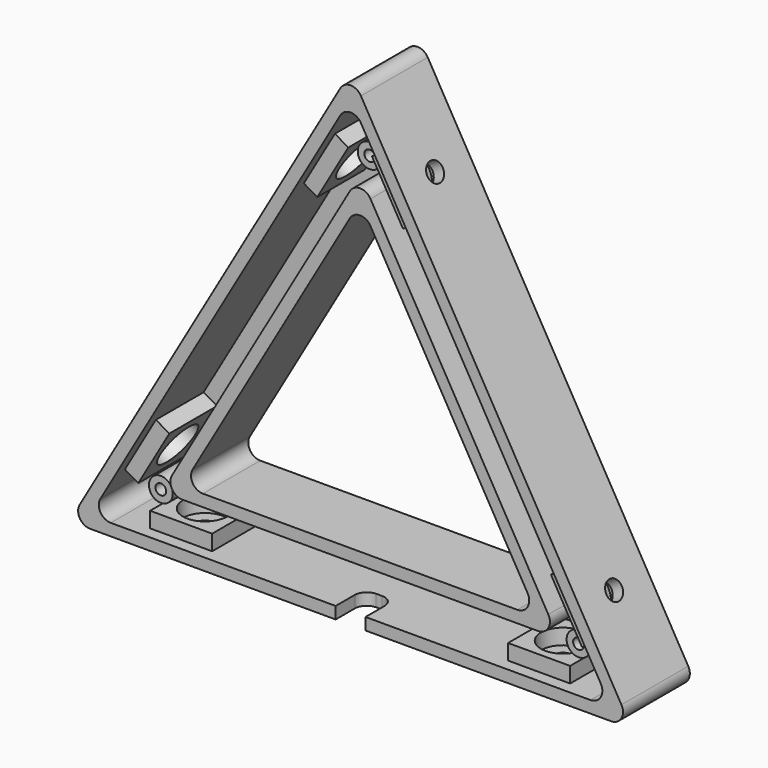
from build123d import *

# Parameters (mm, degrees)
F1_DEPTH  = 2
F3_DEPTH  = 12
F5_DEPTH  = 10
F6_R      = 2
F7_W      = 10.4
F7_H      = 2.6
F8_DEPTH  = 10
F9_W      = 5
F9_H      = 6
F9_R      = 1.6
F10_DEPTH = 5
F11_R     = 1.6
F12_DEPTH = 5
F13_R     = 1.6
F14_DEPTH = 5
F15_R     = 2
F16_R     = 3.7
F17_DEPTH = 2.6
F18_R     = 3.7
F19_DEPTH = 2.6
F20_R     = 3.7
F21_DEPTH = 2.6
F22_R     = 2
F22_R_2   = 0.9
F23_DEPTH = 8


# Not quite as in the source:
# - a feature names something its author has since deleted; it is built from what else it names


with BuildPart() as f1:
    # F0 (on Front) → F1 (new body)
    with BuildSketch(Plane.XZ):
        Polygon((47.128, -40.814), (0, 40.8140904591), (-47.128, -40.814), align=None)
        Polygon((-29.8074919243, -30.814), (0, 20.8140904591), (29.8074919243, -30.814), align=None, mode=Mode.SUBTRACT)
    extrude(amount=F1_DEPTH)

    # F2 (on face) → F3 (join)
    with BuildSketch(Plane.XZ.offset(2)):
        Polygon((0, 40.8140904591), (-47.128, -40.814), (47.128, -40.814), align=None)
        Polygon((43.6638983849, -38.814), (-43.6638983849, -38.814), (0, 36.8140904591), align=None, mode=Mode.SUBTRACT)
    extrude(amount=F3_DEPTH)

    # F4 (on face) → F5 (join)
    with BuildSketch(Plane.XZ.offset(2)):
        Polygon((33.2715935394, -32.814), (0, 24.8140904591), (-33.2715935394, -32.814), align=None)
        Polygon((-29.8074919243, -30.814), (0, 20.8140904591), (29.8074919243, -30.814), align=None, mode=Mode.SUBTRACT)
    extrude(amount=F5_DEPTH)

    # F6
    f6_edges = [f1.edges().sort_by_distance(p)[0] for p in [
        (47.128, -7, -40.814),
        (-47.128, -7, -40.814),
        (0, -7, 40.81409),
        (-29.807492, -6, -30.814),
        (-43.663898, -8, -38.814),
        (0, -7, 24.81409),
        (0, -6, 20.81409),
        (0, -8, 36.81409),
        (33.271594, -7, -32.814),
        (-33.271594, -7, -32.814),
        (29.807492, -6, -30.814),
        (43.663898, -8, -38.814),
    ]]
    fillet(f6_edges, radius=F6_R)

    # F7 (on face) → F8 (join)
    with BuildSketch(Plane.XZ.offset(2)):
        Polygon((-31.9803847577, -23.7775607869), (-34.2320508076, -22.4775607869), (-39.4320508076, -31.4842249862), (-37.1803847577, -32.7842249862), align=None)
        Polygon((-9.4320508076, 20.4772992408), (-7.1803847577, 19.1772992408), (-1.9803847577, 28.1839634402), (-4.2320508076, 29.4839634402), align=None)
        Polygon((9.4320508076, 20.4772992408), (4.2320508076, 29.4839634402), (1.9803847577, 28.1839634402), (7.1803847577, 19.1772992408), align=None)
        Polygon((39.4320508076, -31.4842249862), (34.2320508076, -22.4775607869), (31.9803847577, -23.7775607869), (37.1803847577, -32.7842249862), align=None)
        with Locations((29.9997967697, -37.514)):
            Rectangle(F7_W, F7_H)
        with Locations((-30.0002032303, -37.514)):
            Rectangle(F7_W, F7_H)
    extrude(amount=F8_DEPTH)

    # F9 (on face) → F10 (cut)
    with BuildSketch(Plane(origin=(0, 0, -40.814), x_dir=(1, 0, 0), z_dir=(0, 0, -1))):
        with Locations((0, 11)):
            Rectangle(F9_W, F9_H)
        with Locations((-30.0002032303, 7)):
            Circle(F9_R)
        with Locations((29.9997967697, 7)):
            Circle(F9_R)
    extrude(amount=-F10_DEPTH, mode=Mode.SUBTRACT)

    # F11 (on face) → F12 (cut)
    with BuildSketch(Plane(origin=(17.673019585, 0, 10.2035226148), x_dir=(0, 1, 0), z_dir=(0.8660254038, 0, 0.5))):
        with Locations((-7, 18.2178359397)):
            Circle(F11_R)
        with Locations((-7, -41.7821640603)):
            Circle(F11_R)
    extrude(amount=-F12_DEPTH, mode=Mode.SUBTRACT)

    # F13 (on face) → F14 (cut)
    with BuildSketch(Plane(origin=(-17.673019585, 0, 10.2035226148), x_dir=(0, -1, 0), z_dir=(-0.8660254038, 0, 0.5))):
        with Locations((7, 18.2178359397)):
            Circle(F13_R)
        with Locations((7, -41.7821640603)):
            Circle(F13_R)
    extrude(amount=-F14_DEPTH, mode=Mode.SUBTRACT)

    # F15
    f15_edges = [f1.edges().sort_by_distance(p)[0] for p in [
        (-2.5, -8, -39.814),
        (2.5, -8, -39.814),
    ]]
    fillet(f15_edges, radius=F15_R)

    # F16 (on face) → F17 (cut)
    with BuildSketch(Plane.XY.offset(-36.214)):
        with Locations((29.9997967697, -7)):
            Circle(F16_R)
        with Locations((-30.0002032303, -7)):
            Circle(F16_R)
    extrude(amount=-F17_DEPTH, mode=Mode.SUBTRACT)

    # F18 (on face) → F19 (cut)
    with BuildSketch(Plane(origin=(13.6893027276, 0, 7.9035226148), x_dir=(0, -1, 0), z_dir=(-0.8660254038, 0, -0.5))):
        with Locations((7, -41.7821640603)):
            Circle(F18_R)
        with Locations((7, 18.2178359397)):
            Circle(F18_R)
    extrude(amount=-F19_DEPTH, mode=Mode.SUBTRACT)

    # F20 (on face) → F21 (cut)
    with BuildSketch(Plane(origin=(-13.6893027276, 0, 7.9035226148), x_dir=(0, 1, 0), z_dir=(0.8660254038, 0, -0.5))):
        with Locations((-7, -41.7821640603)):
            Circle(F20_R)
        with Locations((-7, 18.2178359397)):
            Circle(F20_R)
    extrude(amount=-F21_DEPTH, mode=Mode.SUBTRACT)

    # F22 (on face) → F23 (join)
    with BuildSketch(Plane.XZ.offset(2)):
        with Locations((0, 26.8140904591)):
            Circle(F22_R)
        with Locations((0, 26.8140904591)):
            Circle(F22_R_2, mode=Mode.SUBTRACT)
        with Locations((35.003644347, -33.814)):
            Circle(F22_R)
        with Locations((35.003644347, -33.814)):
            Circle(F22_R_2, mode=Mode.SUBTRACT)
        with Locations((-35.003644347, -33.814)):
            Circle(F22_R)
        with Locations((-35.003644347, -33.814)):
            Circle(F22_R_2, mode=Mode.SUBTRACT)
    extrude(amount=F23_DEPTH)


solid = f1.part
